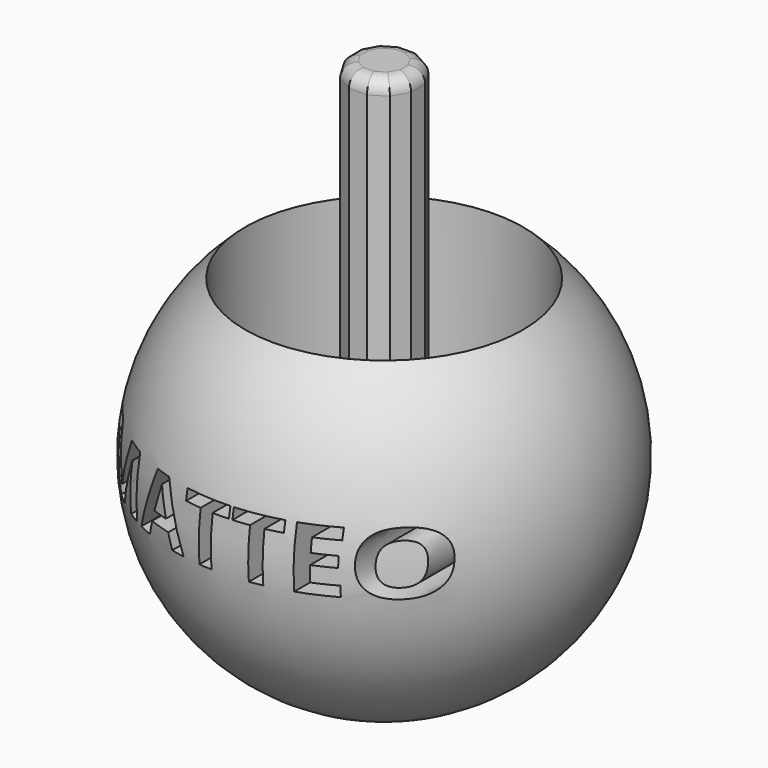
from build123d import *

# Parameters (mm, degrees)
F2_R         = 10
F3_DEPTH     = 15.001
F5_DEPTH     = 25
F6_R         = 1
F8_TEXT_SIZE = 6.0188842493
F9_DEPTH     = 22


# Not quite as in the source:
# - Text() gives the source's letters only with a copy of the font that has no kerning and outlines rounded to 1/6400 em; it was checked with that copy


with BuildPart() as f1:
    # F0 (on Front) → F1 (revolve)
    with BuildSketch(Plane.XZ):
        with BuildLine():
            ThreePointArc((0, -15), (10.6066017178, -10.6066017178), (15, 0))
            ThreePointArc((15, 0), (10.6066017178, 10.6066017178), (0, 15))
            Line((0, 15), (0, -15))
        make_face()
    revolve(axis=Axis((0, 0, 0), (0, 0, -1)))

    # F2 (on Top) → F3 (cut, through all)
    with BuildSketch(Plane.XY):
        Circle(F2_R)
    extrude(amount=F3_DEPTH, mode=Mode.SUBTRACT)

    # F4 (on face) → F5 (join)
    with BuildSketch(Plane.XY):
        Polygon((2.4034209325, 0.6881626416), (1.7373422627, 1.7976767958), (0.6057441367, 2.4255049043), (-0.6881626416, 2.4034209325), (-1.7976767958, 1.7373422627), (-2.4255049043, 0.6057441367), (-2.4034209325, -0.6881626416), (-1.7373422627, -1.7976767958), (-0.6057441367, -2.4255049043), (0.6881626416, -2.4034209325), (1.7976767958, -1.7373422627), (2.4255049043, -0.6057441367), align=None)
    extrude(amount=F5_DEPTH)

    # F6
    f6_edges = [f1.edges().sort_by_distance(p)[0] for p in [
        (0.041209, -2.414463, 25),
        (1.24292, -2.070382, 25),
        (2.111591, -1.171543, 25),
        (2.414463, 0.041209, 25),
        (2.070382, 1.24292, 25),
        (1.171543, 2.111591, 25),
        (-0.041209, 2.414463, 25),
        (-1.24292, 2.070382, 25),
        (-2.111591, 1.171543, 25),
        (-2.414463, -0.041209, 25),
        (-2.070382, -1.24292, 25),
        (-1.171543, -2.111591, 25),
    ]]
    fillet(f6_edges, radius=F6_R)

    # F8 (on offset) → F9 (cut)
    with BuildSketch(Plane.XZ.offset(25)):
        with Locations((-12.5, -1.3335966595)):
            Text('MATTEO', F8_TEXT_SIZE, font='Open Sans', font_style=FontStyle.BOLD, text_align=(TextAlign.LEFT, TextAlign.BOTTOM))
    extrude(amount=-F9_DEPTH, mode=Mode.SUBTRACT)


solid = f1.part
